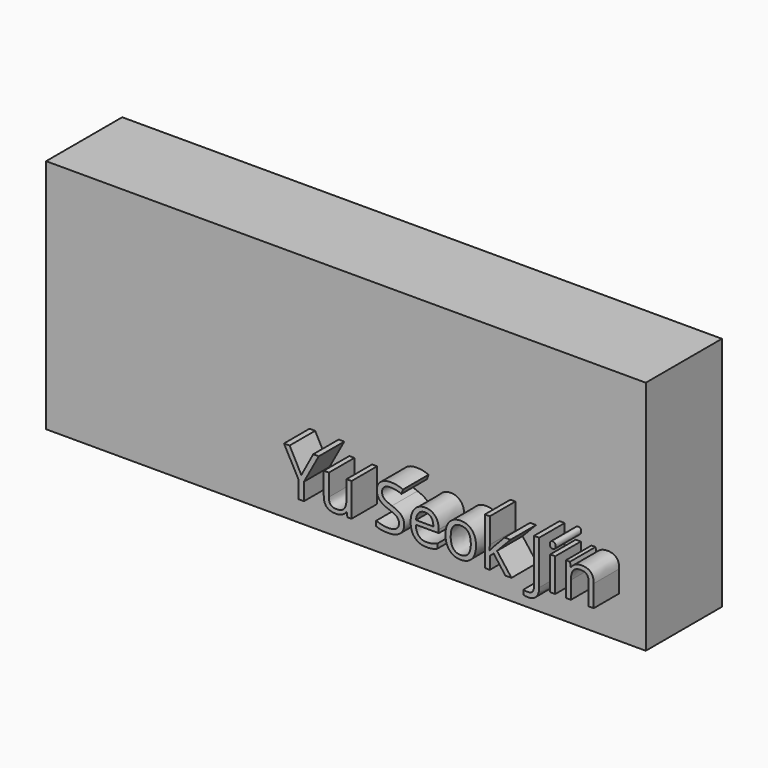
from build123d import *

# Parameters (mm, degrees)
F0_W         = 93.9287915826
F0_H         = 36.9631461799
F1_DEPTH     = 9.906
F2_TEXT_SIZE = 9.7298373779
F1_FACE1_W   = 93.9287915826
F1_FACE1_H   = 36.9631461799
F3_DEPTH     = 5
F4_W         = 93.9287915826
F4_H         = 36.9631461799
F4_W_2       = 2.3514242442
F4_H_2       = 0.7281137653
F4_TEXT_SIZE = 9.8103749432
F5_DEPTH     = 5
F6_DEPTH     = 5


# Not quite as in the source:
# - Text() gives the source's letters only with a copy of the font that has no kerning and outlines rounded to 1/6400 em; it was checked with that copy


with BuildPart() as f1:
    # F0 (on Front) → F1 (new body)
    with BuildSketch(Plane.XZ):
        with Locations((46.9643957913, 18.48157309)):
            Rectangle(F0_W, F0_H)
    extrude(amount=F1_DEPTH)

    # F2 (on face) + F1_face1 (on face) → F3 (join)
    with BuildSketch(Plane.XZ.offset(9.906)):
        with Locations((41.2596960038, 6.5445965156)):
            Text('Yu Seok Jin', F2_TEXT_SIZE, font='Open Sans', text_align=(TextAlign.LEFT, TextAlign.BOTTOM))
    with BuildSketch(Plane(origin=(46.9643957913, 0, 18.48157309), x_dir=(1, 0, 0), z_dir=(0, 1, 0))):
        Rectangle(F1_FACE1_W, F1_FACE1_H)
    extrude(amount=F3_DEPTH, dir=(0, -1, 0))

    # F4 (on face) → F5 (join)
    with BuildSketch(Plane(origin=(0, 0, 0), x_dir=(-1, 0, 0), z_dir=(0, 1, 0))):
        with Locations((-46.9643957913, 18.48157309)):
            Rectangle(F4_W, F4_H)
        with BuildLine():
            add(Edge.make_bspline(
                [(-63.5405722102, 14.0078784503), (-62.9488839714, 13.0827907505), (-62.9488839714, 11.3307191005)],
                knots=[0, 0, 0, 1, 1, 1], degree=2))
            add(Edge.make_bspline(
                [(-62.9488839714, 11.3307191005), (-62.9488839714, 9.514266865), (-63.5214113216, 8.6183037159)],
                knots=[0, 0, 0, 1, 1, 1], degree=2))
            add(Edge.make_bspline(
                [(-63.5214113216, 8.6183037159), (-64.0939386718, 7.7223405667), (-65.2727165361, 7.7223405667)],
                knots=[0, 0, 0, 1, 1, 1], degree=2))
            add(Edge.make_bspline(
                [(-65.2727165361, 7.7223405667), (-66.4024425256, 7.7223405667), (-66.9918314577, 8.639763911)],
                knots=[0, 0, 0, 1, 1, 1], degree=2))
            add(Edge.make_bspline(
                [(-66.9918314577, 8.639763911), (-67.5812203899, 9.5571872553), (-67.5812203899, 11.3307191005)],
                knots=[0, 0, 0, 1, 1, 1], degree=2))
            add(Edge.make_bspline(
                [(-67.5812203899, 11.3307191005), (-67.5812203899, 13.1594343048), (-67.0109923463, 14.0462002274)],
                knots=[0, 0, 0, 1, 1, 1], degree=2))
            add(Edge.make_bspline(
                [(-67.0109923463, 14.0462002274), (-66.4407643027, 14.93296615), (-65.2727165361, 14.93296615)],
                knots=[0, 0, 0, 1, 1, 1], degree=2))
            add(Edge.make_bspline(
                [(-65.2727165361, 14.93296615), (-64.1322604489, 14.93296615), (-63.5405722102, 14.0078784503)],
                knots=[0, 0, 0, 1, 1, 1], degree=2))
        make_face(mode=Mode.SUBTRACT)
        with BuildLine():
            Line((-59.0369969628, 14.8225994319), (-59.0369969628, 7.8189114451))
            Line((-59.0369969628, 7.8189114451), (-59.8126297317, 7.8189114451))
            Line((-59.8126297317, 7.8189114451), (-59.8126297317, 12.8099396974))
            add(Edge.make_bspline(
                [(-59.8126297317, 12.8099396974), (-59.8126297317, 13.433818229), (-59.7743079546, 13.9887175617)],
                knots=[0, 0, 0, 1, 1, 1], degree=2))
            add(Edge.make_bspline(
                [(-59.7743079546, 13.9887175617), (-59.8739445751, 13.8875480701), (-59.9988735686, 13.7779477875)],
                knots=[0, 0, 0, 1, 1, 1], degree=2))
            add(Edge.make_bspline(
                [(-59.9988735686, 13.7779477875), (-60.123802562, 13.668347505), (-61.1385632202, 12.8436628613)],
                knots=[0, 0, 0, 1, 1, 1], degree=2))
            Line((-61.1385632202, 12.8436628613), (-61.5601027685, 13.3893649675))
            Line((-61.5601027685, 13.3893649675), (-59.7068616269, 14.8225994319))
            Line((-59.7068616269, 14.8225994319), (-59.0369969628, 14.8225994319))
        make_face(mode=Mode.SUBTRACT)
        with BuildLine():
            add(Edge.make_bspline(
                [(-52.3230216111, 14.0078784503), (-51.7313333723, 13.0827907505), (-51.7313333723, 11.3307191005)],
                knots=[0, 0, 0, 1, 1, 1], degree=2))
            add(Edge.make_bspline(
                [(-51.7313333723, 11.3307191005), (-51.7313333723, 9.514266865), (-52.3038607225, 8.6183037159)],
                knots=[0, 0, 0, 1, 1, 1], degree=2))
            add(Edge.make_bspline(
                [(-52.3038607225, 8.6183037159), (-52.8763880727, 7.7223405667), (-54.055165937, 7.7223405667)],
                knots=[0, 0, 0, 1, 1, 1], degree=2))
            add(Edge.make_bspline(
                [(-54.055165937, 7.7223405667), (-55.1848919265, 7.7223405667), (-55.7742808586, 8.639763911)],
                knots=[0, 0, 0, 1, 1, 1], degree=2))
            add(Edge.make_bspline(
                [(-55.7742808586, 8.639763911), (-56.3636697908, 9.5571872553), (-56.3636697908, 11.3307191005)],
                knots=[0, 0, 0, 1, 1, 1], degree=2))
            add(Edge.make_bspline(
                [(-56.3636697908, 11.3307191005), (-56.3636697908, 13.1594343048), (-55.7934417472, 14.0462002274)],
                knots=[0, 0, 0, 1, 1, 1], degree=2))
            add(Edge.make_bspline(
                [(-55.7934417472, 14.0462002274), (-55.2232137036, 14.93296615), (-54.055165937, 14.93296615)],
                knots=[0, 0, 0, 1, 1, 1], degree=2))
            add(Edge.make_bspline(
                [(-54.055165937, 14.93296615), (-52.9147098498, 14.93296615), (-52.3230216111, 14.0078784503)],
                knots=[0, 0, 0, 1, 1, 1], degree=2))
        make_face(mode=Mode.SUBTRACT)
        with Locations((-49.6650231499, 10.4485517912)):
            Rectangle(F4_W_2, F4_H_2, mode=Mode.SUBTRACT)
        with BuildLine():
            Line((-43.0046982861, 8.5562224369), (-43.0046982861, 7.8189114451))
            Line((-43.0046982861, 7.8189114451), (-47.607910154, 7.8189114451))
            Line((-47.607910154, 7.8189114451), (-47.607910154, 8.50410482))
            Line((-47.607910154, 8.50410482), (-45.7638662389, 10.3573459616))
            add(Edge.make_bspline(
                [(-45.7638662389, 10.3573459616), (-44.9207871422, 11.2111551559), (-44.6525347024, 11.5752120386)],
                knots=[0, 0, 0, 1, 1, 1], degree=2))
            add(Edge.make_bspline(
                [(-44.6525347024, 11.5752120386), (-44.3842822625, 11.9392689212), (-44.2501560426, 12.2841649153)],
                knots=[0, 0, 0, 1, 1, 1], degree=2))
            add(Edge.make_bspline(
                [(-44.2501560426, 12.2841649153), (-44.1160298226, 12.6290609094), (-44.1160298226, 13.0260745204)],
                knots=[0, 0, 0, 1, 1, 1], degree=2))
            add(Edge.make_bspline(
                [(-44.1160298226, 13.0260745204), (-44.1160298226, 13.5871053375), (-44.4563272035, 13.9151397496)],
                knots=[0, 0, 0, 1, 1, 1], degree=2))
            add(Edge.make_bspline(
                [(-44.4563272035, 13.9151397496), (-44.7966245843, 14.2431741618), (-45.4005757918, 14.2431741618)],
                knots=[0, 0, 0, 1, 1, 1], degree=2))
            add(Edge.make_bspline(
                [(-45.4005757918, 14.2431741618), (-45.8359111799, 14.2431741618), (-46.2267933065, 14.0990842798)],
                knots=[0, 0, 0, 1, 1, 1], degree=2))
            add(Edge.make_bspline(
                [(-46.2267933065, 14.0990842798), (-46.6176754332, 13.9549943978), (-47.0959312116, 13.5763752399)],
                knots=[0, 0, 0, 1, 1, 1], degree=2))
            Line((-47.0959312116, 13.5763752399), (-47.51747076, 14.1174787328))
            add(Edge.make_bspline(
                [(-47.51747076, 14.1174787328), (-46.5502291054, 14.9222360524), (-45.4097730183, 14.9222360524)],
                knots=[0, 0, 0, 1, 1, 1], degree=2))
            add(Edge.make_bspline(
                [(-45.4097730183, 14.9222360524), (-44.4226040396, 14.9222360524), (-43.8623396581, 14.4171550299)],
                knots=[0, 0, 0, 1, 1, 1], degree=2))
            add(Edge.make_bspline(
                [(-43.8623396581, 14.4171550299), (-43.3020752766, 13.9120740075), (-43.3020752766, 13.0597976843)],
                knots=[0, 0, 0, 1, 1, 1], degree=2))
            add(Edge.make_bspline(
                [(-43.3020752766, 13.0597976843), (-43.3020752766, 12.3929987624), (-43.6760958213, 11.7415285513)],
                knots=[0, 0, 0, 1, 1, 1], degree=2))
            add(Edge.make_bspline(
                [(-43.6760958213, 11.7415285513), (-44.050116366, 11.0900583402), (-45.0740742507, 10.093692135)],
                knots=[0, 0, 0, 1, 1, 1], degree=2))
            Line((-45.0740742507, 10.093692135), (-46.6069453356, 8.594544214))
            Line((-46.6069453356, 8.594544214), (-46.6069453356, 8.5562224369))
            Line((-46.6069453356, 8.5562224369), (-43.0046982861, 8.5562224369))
        make_face(mode=Mode.SUBTRACT)
        with BuildLine():
            add(Edge.make_bspline(
                [(-41.1882460505, 14.4700390824), (-40.6256823624, 14.9222360524), (-39.6814337741, 14.9222360524)],
                knots=[0, 0, 0, 1, 1, 1], degree=2))
            add(Edge.make_bspline(
                [(-39.6814337741, 14.9222360524), (-38.7233893461, 14.9222360524), (-38.1631249645, 14.4769370022)],
                knots=[0, 0, 0, 1, 1, 1], degree=2))
            add(Edge.make_bspline(
                [(-38.1631249645, 14.4769370022), (-37.602860583, 14.0316379521), (-37.602860583, 13.2468079566)],
                knots=[0, 0, 0, 1, 1, 1], degree=2))
            add(Edge.make_bspline(
                [(-37.602860583, 13.2468079566), (-37.602860583, 12.7286975299), (-37.9232306398, 12.3025593683)],
                knots=[0, 0, 0, 1, 1, 1], degree=2))
            add(Edge.make_bspline(
                [(-37.9232306398, 12.3025593683), (-38.2436006965, 11.8764212068), (-38.9487213955, 11.5269265994)],
                knots=[0, 0, 0, 1, 1, 1], degree=2))
            add(Edge.make_bspline(
                [(-38.9487213955, 11.5269265994), (-38.0964450723, 11.1191828908), (-37.7369868029, 10.671584534)],
                knots=[0, 0, 0, 1, 1, 1], degree=2))
            add(Edge.make_bspline(
                [(-37.7369868029, 10.671584534), (-37.3775285335, 10.2239861773), (-37.3775285335, 9.6338308096)],
                knots=[0, 0, 0, 1, 1, 1], degree=2))
            add(Edge.make_bspline(
                [(-37.3775285335, 9.6338308096), (-37.3775285335, 8.7631600334), (-37.9860783542, 8.2427503001)],
                knots=[0, 0, 0, 1, 1, 1], degree=2))
            add(Edge.make_bspline(
                [(-37.9860783542, 8.2427503001), (-38.5946281749, 7.7223405667), (-39.6523092235, 7.7223405667)],
                knots=[0, 0, 0, 1, 1, 1], degree=2))
            add(Edge.make_bspline(
                [(-39.6523092235, 7.7223405667), (-40.7728379865, 7.7223405667), (-41.376789194, 8.2136257494)],
                knots=[0, 0, 0, 1, 1, 1], degree=2))
            add(Edge.make_bspline(
                [(-41.376789194, 8.2136257494), (-41.9807404014, 8.7049109322), (-41.9807404014, 9.6062391301)],
                knots=[0, 0, 0, 1, 1, 1], degree=2))
            add(Edge.make_bspline(
                [(-41.9807404014, 9.6062391301), (-41.9807404014, 10.8080100606), (-40.5153156443, 11.4794075958)],
                knots=[0, 0, 0, 1, 1, 1], degree=2))
            add(Edge.make_bspline(
                [(-40.5153156443, 11.4794075958), (-41.1759830819, 11.8518952694), (-41.4633964103, 12.2856977864)],
                knots=[0, 0, 0, 1, 1, 1], degree=2))
            add(Edge.make_bspline(
                [(-41.4633964103, 12.2856977864), (-41.7508097387, 12.7195003034), (-41.7508097387, 13.2560051831)],
                knots=[0, 0, 0, 1, 1, 1], degree=2))
            add(Edge.make_bspline(
                [(-41.7508097387, 13.2560051831), (-41.7508097387, 14.0178421123), (-41.1882460505, 14.4700390824)],
                knots=[0, 0, 0, 1, 1, 1], degree=2))
        make_face(mode=Mode.SUBTRACT)
        Polygon((-31.4575804038, 10.1519412363), (-31.4575804038, 9.4284260842), (-32.4968669993, 9.4284260842), (-32.4968669993, 7.8189114451), (-33.2587039285, 7.8189114451), (-33.2587039285, 9.4284260842), (-36.6647434791, 9.4284260842), (-36.6647434791, 10.1228166857), (-33.339946096, 14.860921209), (-32.4968669993, 14.860921209), (-32.4968669993, 10.1519412363), align=None, mode=Mode.SUBTRACT)
        Polygon((-29.0141838945, 7.8189114451), (-29.8955847683, 7.8189114451), (-26.9938598046, 14.0898870533), (-30.8107088059, 14.0898870533), (-30.8107088059, 14.8225994319), (-26.1507807079, 14.8225994319), (-26.1507807079, 14.1849250606), align=None, mode=Mode.SUBTRACT)
        with Locations((-24.0737403879, 10.4485517912)):
            Rectangle(F4_W_2, F4_H_2, mode=Mode.SUBTRACT)
        with BuildLine():
            add(Edge.make_bspline(
                [(-21.2984772888, 8.539360855), (-21.9353852245, 9.3563811432), (-21.9353852245, 10.8126086739)],
                knots=[0, 0, 0, 1, 1, 1], degree=2))
            add(Edge.make_bspline(
                [(-21.9353852245, 10.8126086739), (-21.9353852245, 12.8773860252), (-21.1329272116, 13.8998110388)],
                knots=[0, 0, 0, 1, 1, 1], degree=2))
            add(Edge.make_bspline(
                [(-21.1329272116, 13.8998110388), (-20.3304691987, 14.9222360524), (-18.7592763367, 14.9222360524)],
                knots=[0, 0, 0, 1, 1, 1], degree=2))
            add(Edge.make_bspline(
                [(-18.7592763367, 14.9222360524), (-18.2181728437, 14.9222360524), (-17.9070000135, 14.8317966584)],
                knots=[0, 0, 0, 1, 1, 1], degree=2))
            Line((-17.9070000135, 14.8317966584), (-17.9070000135, 14.1466032835))
            add(Edge.make_bspline(
                [(-17.9070000135, 14.1466032835), (-18.2764219449, 14.2661672281), (-18.7500791102, 14.2661672281)],
                knots=[0, 0, 0, 1, 1, 1], degree=2))
            add(Edge.make_bspline(
                [(-18.7500791102, 14.2661672281), (-19.8767393575, 14.2661672281), (-20.4707269029, 13.5648787067)],
                knots=[0, 0, 0, 1, 1, 1], degree=2))
            add(Edge.make_bspline(
                [(-20.4707269029, 13.5648787067), (-21.0647144483, 12.8635901854), (-21.1214306785, 11.3583107801)],
                knots=[0, 0, 0, 1, 1, 1], degree=2))
            Line((-21.1214306785, 11.3583107801), (-21.0647144483, 11.3583107801))
            add(Edge.make_bspline(
                [(-21.0647144483, 11.3583107801), (-20.5374067951, 12.1829954237), (-19.396950708, 12.1829954237)],
                knots=[0, 0, 0, 1, 1, 1], degree=2))
            add(Edge.make_bspline(
                [(-19.396950708, 12.1829954237), (-18.4527021197, 12.1829954237), (-17.9092993201, 11.6127673802)],
                knots=[0, 0, 0, 1, 1, 1], degree=2))
            add(Edge.make_bspline(
                [(-17.9092993201, 11.6127673802), (-17.3658965205, 11.0425393366), (-17.3658965205, 10.0661004555)],
                knots=[0, 0, 0, 1, 1, 1], degree=2))
            add(Edge.make_bspline(
                [(-17.3658965205, 10.0661004555), (-17.3658965205, 8.973163372), (-17.9621833725, 8.3477519694)],
                knots=[0, 0, 0, 1, 1, 1], degree=2))
            add(Edge.make_bspline(
                [(-17.9621833725, 8.3477519694), (-18.5584702246, 7.7223405667), (-19.5747637538, 7.7223405667)],
                knots=[0, 0, 0, 1, 1, 1], degree=2))
            add(Edge.make_bspline(
                [(-19.5747637538, 7.7223405667), (-20.661569353, 7.7223405667), (-21.2984772888, 8.539360855)],
                knots=[0, 0, 0, 1, 1, 1], degree=2))
        make_face(mode=Mode.SUBTRACT)
        with BuildLine():
            Line((-11.8046402246, 8.5562224369), (-11.8046402246, 7.8189114451))
            Line((-11.8046402246, 7.8189114451), (-16.4078520925, 7.8189114451))
            Line((-16.4078520925, 7.8189114451), (-16.4078520925, 8.50410482))
            Line((-16.4078520925, 8.50410482), (-14.5638081774, 10.3573459616))
            add(Edge.make_bspline(
                [(-14.5638081774, 10.3573459616), (-13.7207290807, 11.2111551559), (-13.4524766408, 11.5752120386)],
                knots=[0, 0, 0, 1, 1, 1], degree=2))
            add(Edge.make_bspline(
                [(-13.4524766408, 11.5752120386), (-13.184224201, 11.9392689212), (-13.0500979811, 12.2841649153)],
                knots=[0, 0, 0, 1, 1, 1], degree=2))
            add(Edge.make_bspline(
                [(-13.0500979811, 12.2841649153), (-12.9159717611, 12.6290609094), (-12.9159717611, 13.0260745204)],
                knots=[0, 0, 0, 1, 1, 1], degree=2))
            add(Edge.make_bspline(
                [(-12.9159717611, 13.0260745204), (-12.9159717611, 13.5871053375), (-13.256269142, 13.9151397496)],
                knots=[0, 0, 0, 1, 1, 1], degree=2))
            add(Edge.make_bspline(
                [(-13.256269142, 13.9151397496), (-13.5965665228, 14.2431741618), (-14.2005177303, 14.2431741618)],
                knots=[0, 0, 0, 1, 1, 1], degree=2))
            add(Edge.make_bspline(
                [(-14.2005177303, 14.2431741618), (-14.6358531184, 14.2431741618), (-15.026735245, 14.0990842798)],
                knots=[0, 0, 0, 1, 1, 1], degree=2))
            add(Edge.make_bspline(
                [(-15.026735245, 14.0990842798), (-15.4176173717, 13.9549943978), (-15.8958731501, 13.5763752399)],
                knots=[0, 0, 0, 1, 1, 1], degree=2))
            Line((-15.8958731501, 13.5763752399), (-16.3174126985, 14.1174787328))
            add(Edge.make_bspline(
                [(-16.3174126985, 14.1174787328), (-15.3501710439, 14.9222360524), (-14.2097149568, 14.9222360524)],
                knots=[0, 0, 0, 1, 1, 1], degree=2))
            add(Edge.make_bspline(
                [(-14.2097149568, 14.9222360524), (-13.2225459781, 14.9222360524), (-12.6622815966, 14.4171550299)],
                knots=[0, 0, 0, 1, 1, 1], degree=2))
            add(Edge.make_bspline(
                [(-12.6622815966, 14.4171550299), (-12.1020172151, 13.9120740075), (-12.1020172151, 13.0597976843)],
                knots=[0, 0, 0, 1, 1, 1], degree=2))
            add(Edge.make_bspline(
                [(-12.1020172151, 13.0597976843), (-12.1020172151, 12.3929987624), (-12.4760377598, 11.7415285513)],
                knots=[0, 0, 0, 1, 1, 1], degree=2))
            add(Edge.make_bspline(
                [(-12.4760377598, 11.7415285513), (-12.8500583045, 11.0900583402), (-13.8740161892, 10.093692135)],
                knots=[0, 0, 0, 1, 1, 1], degree=2))
            Line((-13.8740161892, 10.093692135), (-15.4068872741, 8.594544214))
            Line((-15.4068872741, 8.594544214), (-15.4068872741, 8.5562224369))
            Line((-15.4068872741, 8.5562224369), (-11.8046402246, 8.5562224369))
        make_face(mode=Mode.SUBTRACT)
        Polygon((-9.0316764321, 7.8189114451), (-9.9130773059, 7.8189114451), (-7.0113523422, 14.0898870533), (-10.8282013435, 14.0898870533), (-10.8282013435, 14.8225994319), (-6.1682732455, 14.8225994319), (-6.1682732455, 14.1849250606), align=None, mode=Mode.SUBTRACT)
        with BuildLine():
            add(Edge.make_bspline(
                [(-1.4163728824, 14.4554768071), (-0.8507434521, 13.9887175617), (-0.8507434521, 13.1747630156)],
                knots=[0, 0, 0, 1, 1, 1], degree=2))
            add(Edge.make_bspline(
                [(-0.8507434521, 13.1747630156), (-0.8507434521, 12.5033654805), (-1.2270633034, 12.0772273189)],
                knots=[0, 0, 0, 1, 1, 1], degree=2))
            add(Edge.make_bspline(
                [(-1.2270633034, 12.0772273189), (-1.6033831548, 11.6510891573), (-2.293175143, 11.5069992753)],
                knots=[0, 0, 0, 1, 1, 1], degree=2))
            Line((-2.293175143, 11.5069992753), (-2.293175143, 11.4686774982))
            add(Edge.make_bspline(
                [(-2.293175143, 11.4686774982), (-1.4500960463, 11.3644422644), (-1.0431187733, 10.932939054)],
                knots=[0, 0, 0, 1, 1, 1], degree=2))
            add(Edge.make_bspline(
                [(-1.0431187733, 10.932939054), (-0.6361415002, 10.5014358436), (-0.6361415002, 9.8024466289)],
                knots=[0, 0, 0, 1, 1, 1], degree=2))
            add(Edge.make_bspline(
                [(-0.6361415002, 9.8024466289), (-0.6361415002, 8.8014818105), (-1.3305321017, 8.2619111886)],
                knots=[0, 0, 0, 1, 1, 1], degree=2))
            add(Edge.make_bspline(
                [(-1.3305321017, 8.2619111886), (-2.0249227031, 7.7223405667), (-3.3033371879, 7.7223405667)],
                knots=[0, 0, 0, 1, 1, 1], degree=2))
            add(Edge.make_bspline(
                [(-3.3033371879, 7.7223405667), (-3.8597693917, 7.7223405667), (-4.3219300238, 7.8066484764)],
                knots=[0, 0, 0, 1, 1, 1], degree=2))
            add(Edge.make_bspline(
                [(-4.3219300238, 7.8066484764), (-4.7840906559, 7.8909563861), (-5.219426044, 8.1009597247)],
                knots=[0, 0, 0, 1, 1, 1], degree=2))
            Line((-5.219426044, 8.1009597247), (-5.219426044, 8.8581980406))
            add(Edge.make_bspline(
                [(-5.219426044, 8.8581980406), (-4.7641633318, 8.6328659912), (-4.2491186473, 8.5156013532)],
                knots=[0, 0, 0, 1, 1, 1], degree=2))
            add(Edge.make_bspline(
                [(-4.2491186473, 8.5156013532), (-3.7340739628, 8.3983367152), (-3.2742126373, 8.3983367152)],
                knots=[0, 0, 0, 1, 1, 1], degree=2))
            add(Edge.make_bspline(
                [(-3.2742126373, 8.3983367152), (-1.4592932728, 8.3983367152), (-1.4592932728, 9.8208410819)],
                knots=[0, 0, 0, 1, 1, 1], degree=2))
            add(Edge.make_bspline(
                [(-1.4592932728, 9.8208410819), (-1.4592932728, 11.0961898246), (-3.4612229096, 11.0961898246)],
                knots=[0, 0, 0, 1, 1, 1], degree=2))
            Line((-3.4612229096, 11.0961898246), (-4.1510148978, 11.0961898246))
            Line((-4.1510148978, 11.0961898246), (-4.1510148978, 11.7798503284))
            Line((-4.1510148978, 11.7798503284), (-3.4520256831, 11.7798503284))
            add(Edge.make_bspline(
                [(-3.4520256831, 11.7798503284), (-2.6334725238, 11.7798503284), (-2.1544503098, 12.1416079044)],
                knots=[0, 0, 0, 1, 1, 1], degree=2))
            add(Edge.make_bspline(
                [(-2.1544503098, 12.1416079044), (-1.6754280958, 12.5033654805), (-1.6754280958, 13.145638465)],
                knots=[0, 0, 0, 1, 1, 1], degree=2))
            add(Edge.make_bspline(
                [(-1.6754280958, 13.145638465), (-1.6754280958, 13.6576174074), (-2.0272220097, 13.9503957846)],
                knots=[0, 0, 0, 1, 1, 1], degree=2))
            add(Edge.make_bspline(
                [(-2.0272220097, 13.9503957846), (-2.3790159237, 14.2431741618), (-2.9829671312, 14.2431741618)],
                knots=[0, 0, 0, 1, 1, 1], degree=2))
            add(Edge.make_bspline(
                [(-2.9829671312, 14.2431741618), (-3.4428284566, 14.2431741618), (-3.8498057297, 14.1182451684)],
                knots=[0, 0, 0, 1, 1, 1], degree=2))
            add(Edge.make_bspline(
                [(-3.8498057297, 14.1182451684), (-4.2567830027, 13.993316175), (-4.7794920426, 13.6576174074)],
                knots=[0, 0, 0, 1, 1, 1], degree=2))
            Line((-4.7794920426, 13.6576174074), (-5.1811042669, 14.1941222871))
            add(Edge.make_bspline(
                [(-5.1811042669, 14.1941222871), (-4.750367492, 14.5344196679), (-4.1878038039, 14.7283278602)],
                knots=[0, 0, 0, 1, 1, 1], degree=2))
            add(Edge.make_bspline(
                [(-4.1878038039, 14.7283278602), (-3.6252401157, 14.9222360524), (-3.0013615842, 14.9222360524)],
                knots=[0, 0, 0, 1, 1, 1], degree=2))
            add(Edge.make_bspline(
                [(-3.0013615842, 14.9222360524), (-1.9820023127, 14.9222360524), (-1.4163728824, 14.4554768071)],
                knots=[0, 0, 0, 1, 1, 1], degree=2))
        make_face(mode=Mode.SUBTRACT)
        with Locations((-68.070206266, 7.8189114451)):
            Text('010-2847-6273', F4_TEXT_SIZE, font='Open Sans', text_align=(TextAlign.LEFT, TextAlign.BOTTOM))
    extrude(amount=F5_DEPTH)

    # F4 (on face) → F6 (join)
    with BuildSketch(Plane(origin=(0, 0, 0), x_dir=(-1, 0, 0), z_dir=(0, 1, 0))):
        with Locations((-68.070206266, 7.8189114451)):
            Text('010-2847-6273', F4_TEXT_SIZE, font='Open Sans', text_align=(TextAlign.LEFT, TextAlign.BOTTOM))
    extrude(amount=F6_DEPTH)


solid = f1.part
